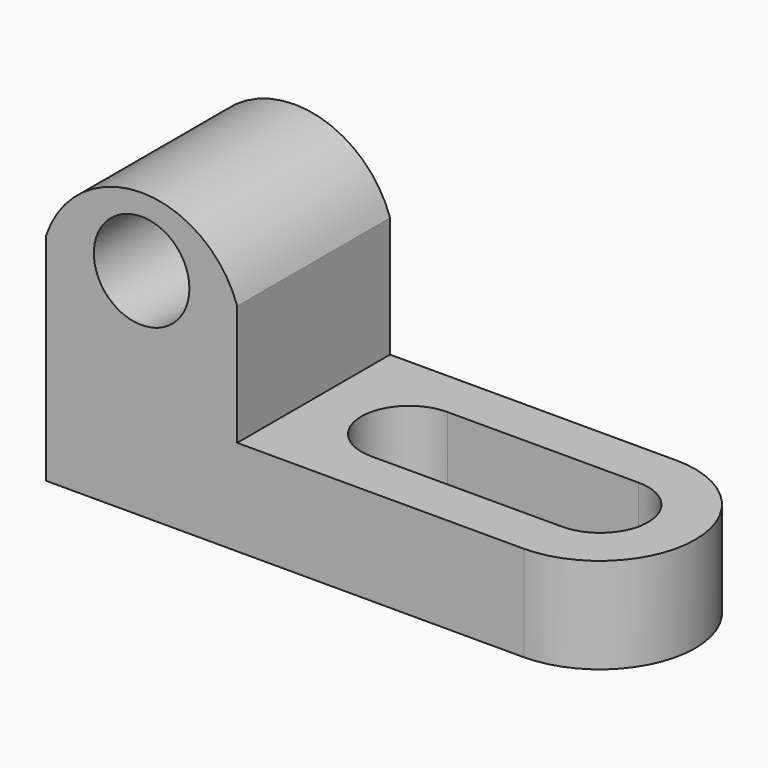
from build123d import *

# Parameters (mm, degrees)
F0_R     = 6.35
F1_DEPTH = 25.4
F3_DEPTH = 25.4
F5_DEPTH = 25.4


with BuildPart() as f1:
    # F0 (on Front) → F1 (new body)
    with BuildSketch(Plane.XZ):
        with BuildLine():
            Line((0, 28.6947377026), (0, 0))
            Line((0, 0), (76.2, 0))
            Line((76.2, 0), (76.2, 12.7))
            Line((76.2, 12.7), (25.4, 12.7))
            Line((25.4, 12.7), (25.4, 28.6947377026))
            ThreePointArc((25.4, 28.6947377026), (12.7, 37.8535239462), (0, 28.6947377026))
        make_face()
        with Locations((12.7, 28.6947377026)):
            Circle(F0_R, mode=Mode.SUBTRACT)
    extrude(amount=F1_DEPTH)

    # F2 (on face) → F3 (cut)
    with BuildSketch(Plane.XY.offset(12.7)):
        with BuildLine():
            ThreePointArc((38.1, -6.3605568116), (42.5901280605, -8.220428751), (44.45, -12.7105568116))
            ThreePointArc((44.45, -12.7105568116), (42.5901280605, -17.2006848721), (38.1, -19.0605568116))
            Line((38.1, -19.0605568116), (38.1, -19.0711169188))
            Line((38.1, -19.0711169188), (63.5052786794, -19.0499978059))
            Line((63.5052786794, -19.0499978059), (63.5, -6.3499994515))
            Line((63.5, -6.3499994515), (38.1, -6.3605568116))
        make_face()
        with BuildLine():
            Line((38.1, -19.0605568116), (38.1, -6.3605568116))
            ThreePointArc((38.1, -6.3605568116), (31.75, -12.7105568116), (38.1, -19.0605568116))
        make_face()
        with BuildLine():
            ThreePointArc((38.1, -19.0605568116), (42.5901280605, -17.2006848721), (44.45, -12.7105568116))
            ThreePointArc((44.45, -12.7105568116), (42.5901280605, -8.220428751), (38.1, -6.3605568116))
            Line((38.1, -6.3605568116), (38.1, -19.0605568116))
        make_face()
        with BuildLine():
            ThreePointArc((69.85, -12.7), (67.9901280605, -8.2098719395), (63.5, -6.35))
            ThreePointArc((63.5, -6.35), (57.1500005485, -12.7026393399), (63.5052786794, -19.0499978059))
            ThreePointArc((63.5052786794, -19.0499978059), (67.9919939678, -17.1882613775), (69.85, -12.7))
        make_face()
    extrude(amount=-F3_DEPTH, mode=Mode.SUBTRACT)

    # F4 (on face) → F5 (cut)
    with BuildSketch(Plane.XY.offset(12.7)):
        with BuildLine():
            ThreePointArc((63.4973606602, 0), (76.1177273109, -12.7), (63.4973606602, -25.4))
            Line((63.4973606602, -25.4), (76.2, -25.4))
            Line((76.2, -25.4), (76.2, 0))
            Line((76.2, 0), (63.4973606602, 0))
        make_face()
    extrude(amount=-F5_DEPTH, mode=Mode.SUBTRACT)


solid = f1.part
